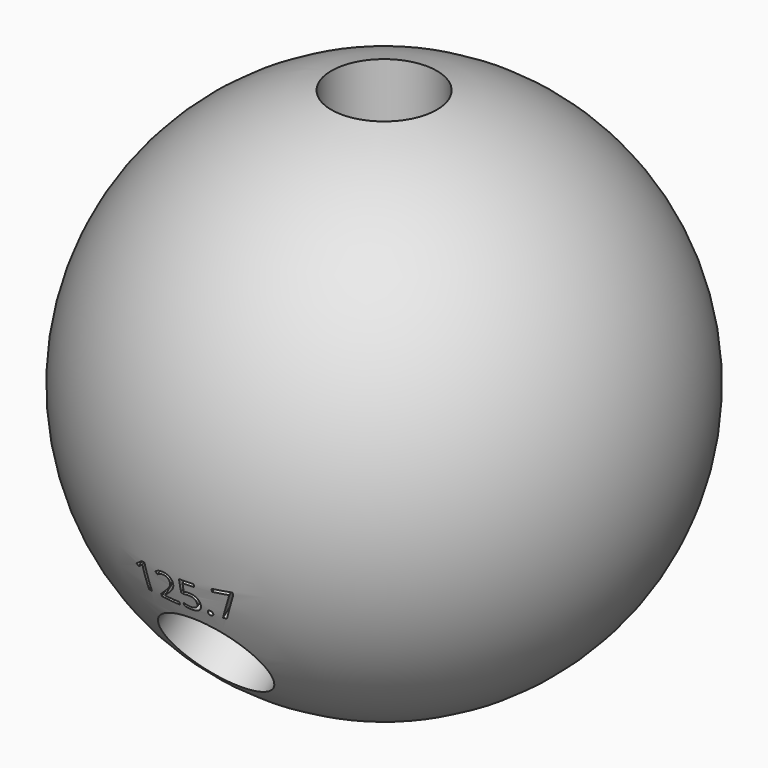
from build123d import *

# Parameters (mm, degrees)
F4_R          = 3.175
F5_DEPTH      = 50.8
F7_ANGLE      = 125.7
F8_ANGLE      = -125.7
F10_TEXT_SIZE = 2.2844602225
F11_DEPTH     = 12.7
F13_TEXT_SIZE = 2.4268655883
F14_DEPTH     = 12.7


# Not quite as in the source:
# - a length typed as a fraction of an inch, garbled in the dataset ("3 / 203.2 mm" for 3/8 in), is restored
# - Text() gives the source's letters only with a copy of the font that has no kerning and outlines rounded to 1/6400 em; it was checked with that copy


with BuildPart() as f2:
    # F0 (on Front) → F2 (revolve)
    with BuildSketch(Plane.XZ):
        with BuildLine():
            Line((0, -15.875), (0, 15.875))
            ThreePointArc((0, 15.875), (-15.875, 0), (0, -15.875))
        make_face()
    revolve(axis=Axis((0, 0, 0), (0, 0, 1)))

    # F10 (on offset) → F11 (cut)
    with BuildSketch(Plane(origin=(0, 15.4701911873, -11.1164600763), x_dir=(-1, 0, 0), z_dir=(0, 0.8120835269, -0.5835412114))):
        with Locations((-2.9321403902, 3.8422925863)):
            Text('125.7', F10_TEXT_SIZE, font='Open Sans', text_align=(TextAlign.LEFT, TextAlign.BOTTOM))
    extrude(amount=-F11_DEPTH, mode=Mode.SUBTRACT)

    # F13 (on offset) → F14 (cut)
    with BuildSketch(Plane(origin=(0, -15.4701911873, -11.1164600763), x_dir=(1, 0, 0), z_dir=(0, -0.8120835269, -0.5835412114))):
        with Locations((-3.1149199023, 3.8645216264)):
            Text('125.7', F13_TEXT_SIZE, font='Open Sans', text_align=(TextAlign.LEFT, TextAlign.BOTTOM))
    extrude(amount=-F14_DEPTH, mode=Mode.SUBTRACT)


with BuildPart() as f5:
    # F4 (on offset) → F5 (new body)
    with BuildSketch(Plane.XY.offset(6.35)):
        Circle(F4_R)
    extrude(amount=F5_DEPTH)


with BuildPart() as f7_1:
    # F7: copy of F5
    add(f5.part.rotate(Axis((29.0340390056, 0, 0), (1, 0, 0)), F7_ANGLE))


with BuildPart() as f8_1:
    # F8: copy of F5
    add(f5.part.rotate(Axis((29.0340390056, 0, 0), (1, 0, 0)), F8_ANGLE))


with BuildPart() as f2_1:
    add(f2.part)

    # F15: cut F5, F7_1, F8_1
    add(f5.part, mode=Mode.SUBTRACT)
    add(f7_1.part, mode=Mode.SUBTRACT)
    add(f8_1.part, mode=Mode.SUBTRACT)


with BuildPart() as f16_1:
    # F16: copy of F2
    add(f2_1.part)


with BuildPart() as f18_1:
    # F18: copy of F2
    add(f2_1.part)


solid = f2_1.part
